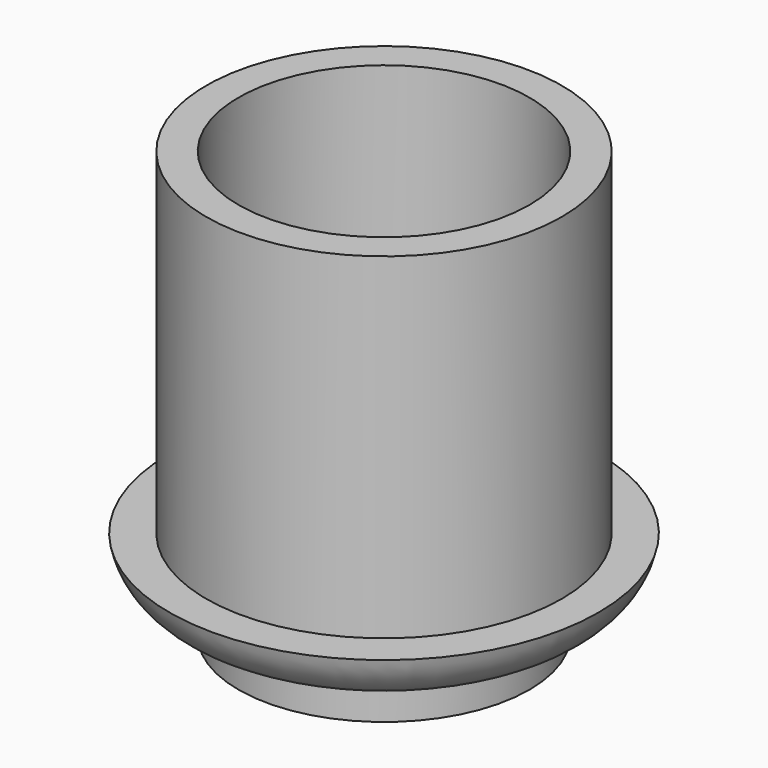
from build123d import *

# Parameters (mm, degrees)
F0_R     = 13.75
F0_R_2   = 11.25
F1_DEPTH = 30
F0_R_3   = 16.6
F2_DEPTH = 4
F4_DEPTH = 3


# Not quite as in the source:
# - a fillet or chamfer that OpenCascade refuses, or shapes differently, is made with other operations: its cross-section is extruded or revolved along the edge and cut away or added


with BuildPart() as f1:
    # F0 (on Top) → F1 (new body)
    with BuildSketch(Plane.XY):
        Circle(F0_R)
        Circle(F0_R_2, mode=Mode.SUBTRACT)
    extrude(amount=F1_DEPTH)

    # F0 (on Top) → F2 (join)
    with BuildSketch(Plane.XY):
        Circle(F0_R_3)
        Circle(F0_R, mode=Mode.SUBTRACT)
    extrude(amount=F2_DEPTH)

    # F3: fillet of radius 5 on 1 edges, made by hand

    # F3_s1 → F3_t2 (revolve, cut)
    with BuildSketch(Plane.XZ):
        with BuildLine():
            ThreePointArc((16.6, 4), (14.8632981746, 1.1270166538), (11.7010205144, 0))
            Line((11.7010205144, 0), (16.6, 0))
            Line((16.6, 0), (16.6, 4))
        make_face()
    revolve(axis=Axis((0, 0, 0), (0, 0, 1)), mode=Mode.SUBTRACT)


with BuildPart() as f4:
    # F0 (on Top) → F4 (new body)
    with BuildSketch(Plane.XY):
        Circle(F0_R_2)
    extrude(amount=-F4_DEPTH)


solid = Compound([f1.part, f4.part])
